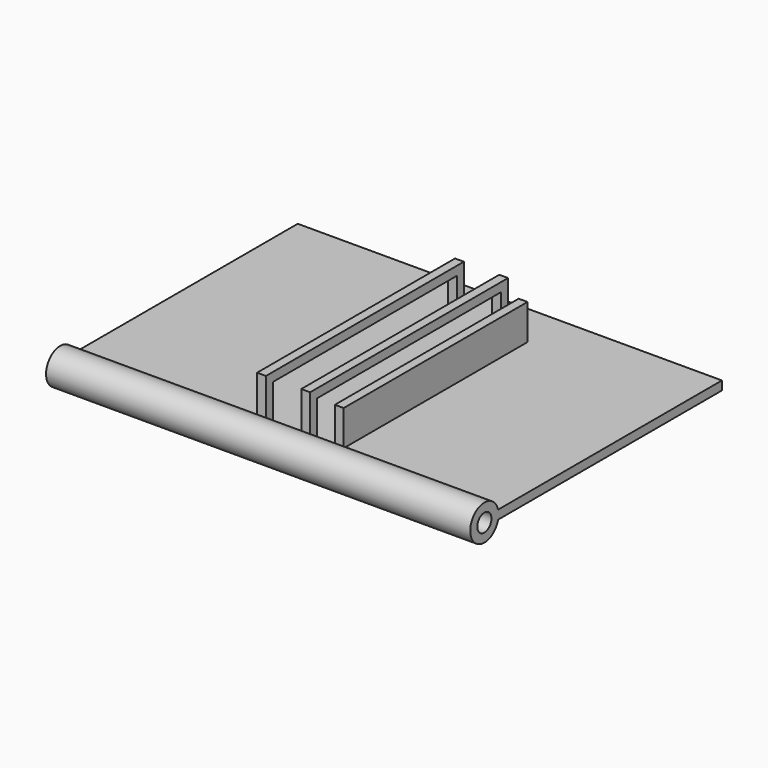
from build123d import *

# Parameters (mm, degrees)
F0_W      = 152.4
F0_H      = 101.6
F1_DEPTH  = 3.175
F2_R      = 6.35
F3_DEPTH  = 76.2
F4_DEPTH  = 76.2
F5_R      = 3.175
F6_DEPTH  = 152.4
F10_DEPTH = 3.175
F13_DEPTH = 3.175
F16_DEPTH = 3.175


# Not quite as in the source:
# - a feature names something its author has since deleted; it is built from what else it names


with BuildPart() as f1:
    # F0 (on Top) → F1 (new body)
    with BuildSketch(Plane.XY):
        Rectangle(F0_W, F0_H)
    extrude(amount=F1_DEPTH)

    # F2 (on Right) → F3 (join)
    with BuildSketch(Plane.YZ):
        with Locations((-55.88, 1.5875)):
            Circle(F2_R)
    extrude(amount=F3_DEPTH)

    # F4 (add): a face of the model
    f4_faces = [f1.faces().sort_by_distance(p)[0] for p in [
        (0, -56.0567159254, 1.5875),
    ]]
    extrude(f4_faces, amount=F4_DEPTH)

    # F5 (on face) → F6 (cut)
    with BuildSketch(Plane.YZ.offset(76.2)):
        with Locations((-55.88, 1.5875)):
            Circle(F5_R)
    extrude(amount=-F6_DEPTH, mode=Mode.SUBTRACT)

    # F9 (on offset) → F10 (join)
    with BuildSketch(Plane.YZ.offset(6.35)):
        Polygon((-50.8, 3.175), (-47.625, 3.175), (-47.625, 15.875), (34.925, 15.875), (34.925, 3.175), (38.1, 3.175), (38.1, 19.05), (-50.8, 19.05), align=None)
    extrude(amount=F10_DEPTH)

    # F12 (on offset) → F13 (join)
    with BuildSketch(Plane.YZ.offset(-6.35)):
        Polygon((-50.8, 3.175), (-47.625, 3.175), (-47.625, 15.875), (34.925, 15.875), (34.925, 3.175), (38.1, 3.175), (38.1, 19.05), (-50.8, 19.05), align=None)
    extrude(amount=-F13_DEPTH)

    # F15 (on offset) → F16 (join)
    with BuildSketch(Plane.YZ.offset(15.875)):
        Polygon((-47.625, 15.875), (-47.625, 3.175), (-47.3777212979, 3.175), (34.925, 3.175), (34.925, 15.875), align=None)
    extrude(amount=F16_DEPTH)


solid = f1.part
